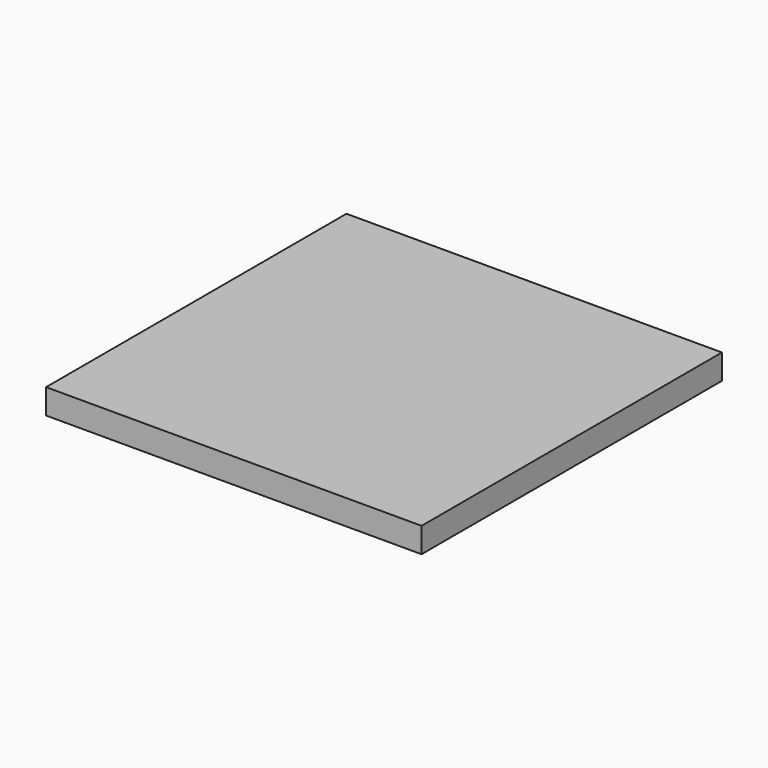
from build123d import *

# Parameters (mm, degrees)
F0_W     = 152.4
F0_H     = 152.4
F3_DEPTH = 5.08


# Not quite as in the source:
# - a feature of the source that left no trace in its solid (it failed there, or was rolled back) is left out


with BuildPart() as f3:
    # F0 (on Top) → F3 (new body, symmetric)
    with BuildSketch(Plane.XY):
        with Locations((-76.2, -76.2)):
            Rectangle(F0_W, F0_H)
    extrude(amount=F3_DEPTH, both=True)


solid = f3.part
